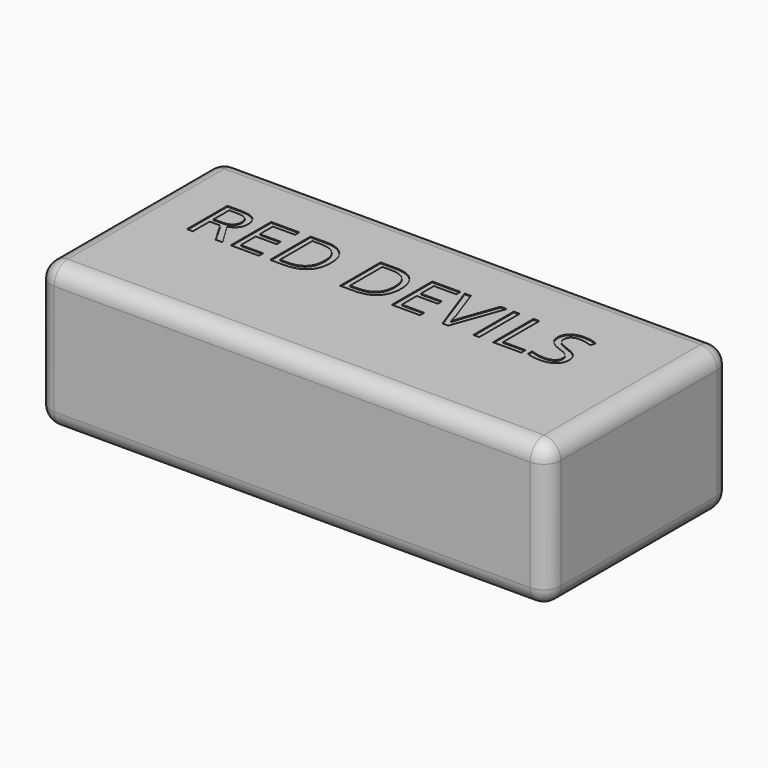
from build123d import *

# Parameters (mm, degrees)
F0_W         = 600
F0_H         = 270
F1_DEPTH     = 170
F2_R         = 20
F3_TEXT_SIZE = 83.3333333333
F4_DEPTH     = 1


# Not quite as in the source:
# - Text() gives the source's letters only with a copy of the font that has no kerning and outlines rounded to 1/6400 em; it was checked with that copy


with BuildPart() as f1:
    # F0 (on Top) → F1 (new body)
    with BuildSketch(Plane.XY):
        Rectangle(F0_W, F0_H)
    extrude(amount=F1_DEPTH)

    # F2
    f2_edges = [f1.edges().sort_by_distance(p)[0] for p in [
        (300, -135, 85),
        (-300, -135, 85),
        (300, 135, 85),
        (0, -135, 0),
        (0, -135, 170),
        (0, 135, 170),
        (300, 0, 0),
        (300, 0, 170),
        (-300, 0, 170),
        (-300, 135, 85),
        (0, 135, 0),
        (-300, 0, 0),
    ]]
    fillet(f2_edges, radius=F2_R)

    # F3 (on face) → F4 (cut)
    with BuildSketch(Plane.XY.offset(170)):
        with Locations((-240, 0)):
            Text('RED DEVILS', F3_TEXT_SIZE, font='Open Sans', text_align=(TextAlign.LEFT, TextAlign.BOTTOM))
    extrude(amount=-F4_DEPTH, mode=Mode.SUBTRACT)


solid = f1.part
